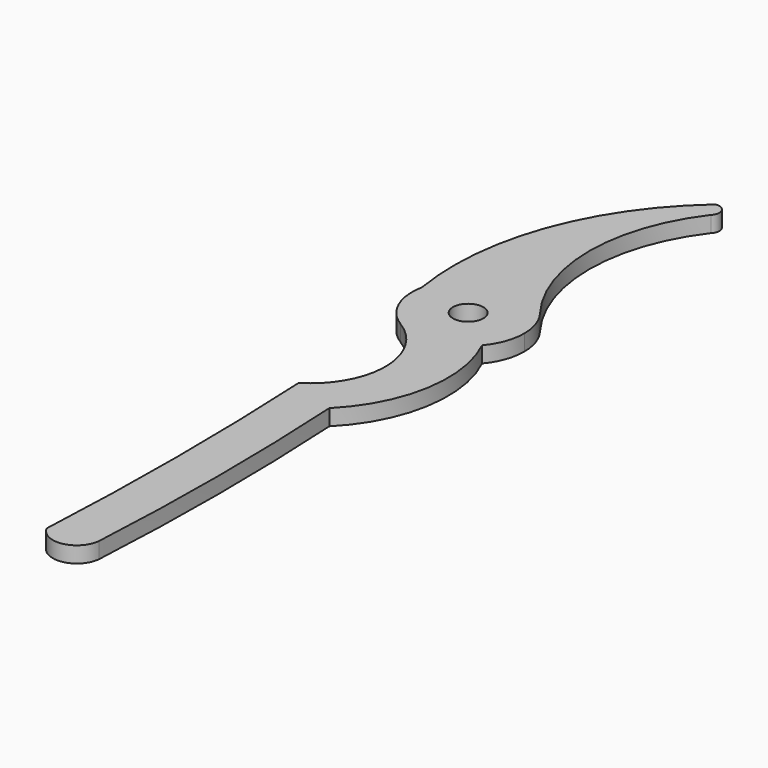
from build123d import *

# Parameters (mm, degrees)
F0_R     = 3.8
F1_DEPTH = 4


# Not quite as in the source:
# - a feature names something its author has since deleted; it is built from what else it names


with BuildPart() as f1:
    # F0 (on Top) → F1 (new body)
    with BuildSketch(Plane.XY):
        with BuildLine():
            ThreePointArc((10.7032142857, -9.0244780433), (13.15, -4.8039046618), (14, 0))
            ThreePointArc((14, 0), (13.2657182303, 4.4744519031), (11.1398971667, 8.4795454545))
            ThreePointArc((11.1398971667, 8.4795454545), (-3.1423826746, 13.6427794502), (-13.7268716756, 2.7519073388))
            ThreePointArc((-13.7268716756, 2.7519073388), (-12.8265756347, -5.610611151), (-7.2967857143, -11.9480926612))
            ThreePointArc((-7.2967857143, -11.9480926612), (-3.7899012351, -13.4772641374), (0, -14))
            ThreePointArc((0, -14), (5.90158061, -12.6953277352), (10.7032142857, -9.0244780433))
        make_face()
        Circle(F0_R, mode=Mode.SUBTRACT)
        with BuildLine():
            ThreePointArc((4.0123564651, -48.3244780433), (13.6087273384, -29.7387061328), (10.7032142857, -9.0244780433))
            ThreePointArc((10.7032142857, -9.0244780433), (5.90158061, -12.6953277352), (0, -14))
            ThreePointArc((0, -14), (-3.7899012351, -13.4772641374), (-7.2967857143, -11.9480926612))
            ThreePointArc((-7.2967857143, -11.9480926612), (1.6235591613, -27.8480926612), (-7.2967857143, -43.7480926612))
            ThreePointArc((-7.2967857143, -43.7480926612), (-6.2932161351, -83.0480926612), (-7.2967857143, -122.3480926612))
            ThreePointArc((-7.2967857143, -122.3480926612), (-0.8068871669, -125.4847000324), (4.0123564651, -120.1244780433))
            ThreePointArc((4.0123564651, -120.1244780433), (5.0200325676, -84.2244780433), (4.0123564651, -48.3244780433))
        make_face()
        with BuildLine():
            ThreePointArc((-13.7268716756, 2.7519073388), (-3.1423826746, 13.6427794502), (11.1398971667, 8.4795454545))
            ThreePointArc((11.1398971667, 8.4795454545), (2.1510025477, 35.1295454545), (11.1398971667, 61.7795454545))
            ThreePointArc((11.1398971667, 61.7795454545), (11.6091204752, 64.5781543581), (9.0255790591, 65.7519073388))
            ThreePointArc((9.0255790591, 65.7519073388), (-10.5763059667, 37.2226044204), (-13.7268716756, 2.7519073388))
        make_face()
    extrude(amount=F1_DEPTH)


solid = f1.part
